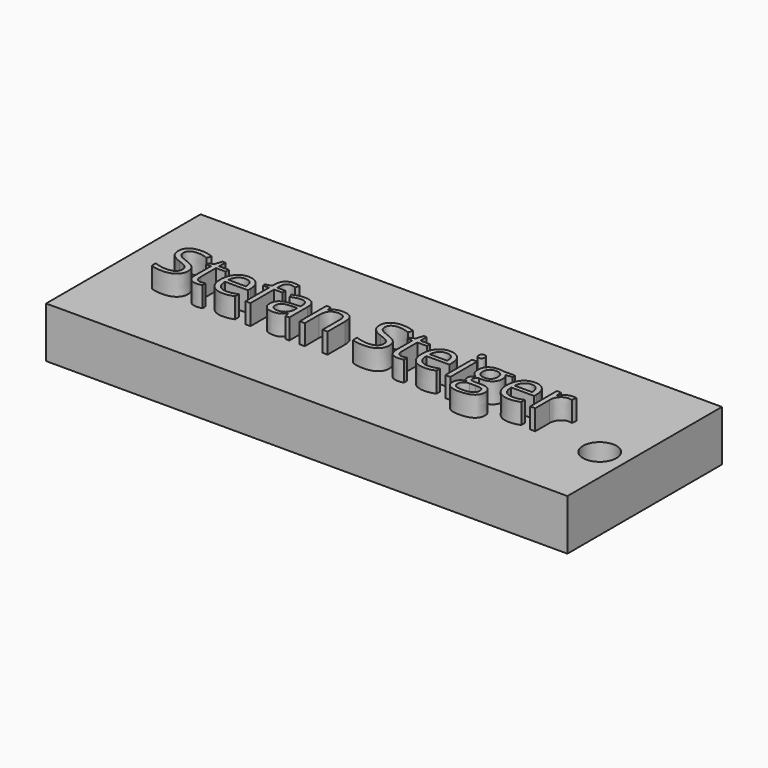
from build123d import *

# Parameters (mm, degrees)
F0_W         = 130.4780244827
F0_H         = 48.3335312456
F0_R         = 4.1792882702
F1_DEPTH     = 12.7
F2_TEXT_SIZE = 15.594033287
F6_DEPTH     = 5.08


# Not quite as in the source:
# - a feature names something its author has since deleted; it is built from what else it names
# - the program builds the solid bodies; features that only make, move or delete a surface that nothing else refers to are left out
# - Text() gives the source's letters only with a copy of the font that has no kerning and outlines rounded to 1/6400 em; it was checked with that copy


with BuildPart() as f1:
    # F0 (on Top) → F1 (new body)
    with BuildSketch(Plane.XY):
        with Locations((36.3598316908, -29.0132844821)):
            Rectangle(F0_W, F0_H)
        with Locations((94.8773249984, -34.6688069403)):
            Circle(F0_R, mode=Mode.SUBTRACT)
    extrude(amount=F1_DEPTH)

    # F2 (on face) → F6 (join)
    with BuildSketch(Plane.XY.offset(12.7)):
        with Locations((-17.4758047833, -35.7165107963)):
            Text('Stefan Steiger', F2_TEXT_SIZE, font='Open Sans', text_align=(TextAlign.LEFT, TextAlign.BOTTOM))
    extrude(amount=F6_DEPTH)


solid = f1.part
